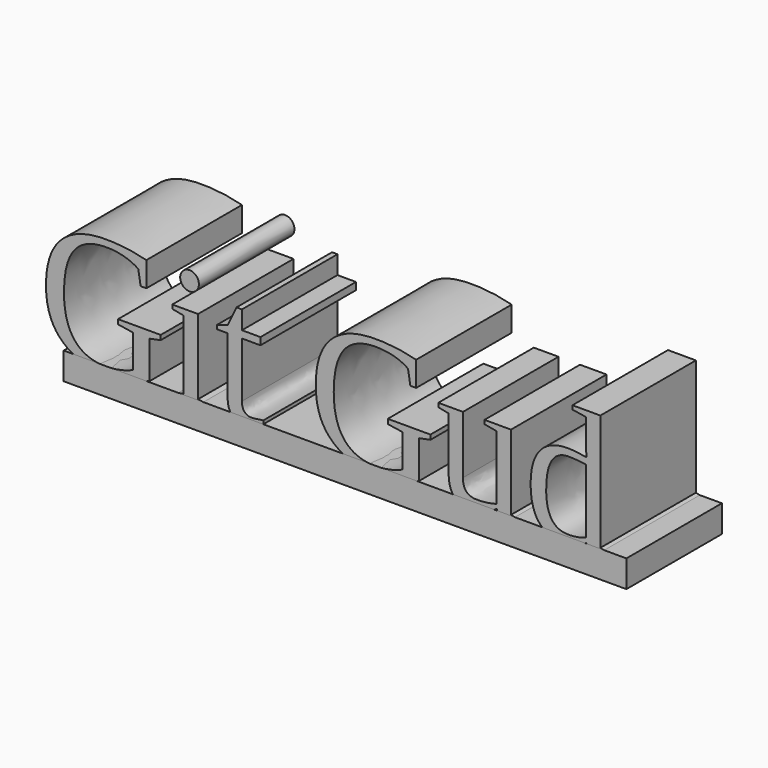
from build123d import *

# Parameters (mm, degrees)
F0_TEXT_SIZE = 37.5547097065
F1_DEPTH     = 25.4
F2_W         = 119.6825578809
F2_H         = 5.7624932379
F3_DEPTH     = 25.4


# Not quite as in the source:
# - Text() gives the source's letters only with a copy of the font that has no kerning and outlines rounded to 1/6400 em; it was checked with that copy


with BuildPart() as f1:
    # F0 (on Front) → F1 (new body)
    with BuildSketch(Plane.XZ):
        with Locations((-64.938865602, -12.1898893267)):
            Text('Git Gud', F0_TEXT_SIZE, font='Tinos', text_align=(TextAlign.LEFT, TextAlign.BOTTOM))
    extrude(amount=F1_DEPTH)


with BuildPart() as f3:
    # F2 (on Front) → F3 (new body)
    with BuildSketch(Plane.XZ):
        with Locations((0.2216361463, -13.9629645273)):
            Rectangle(F2_W, F2_H)
    extrude(amount=F3_DEPTH)


solid = Compound([f1.part, f3.part])
